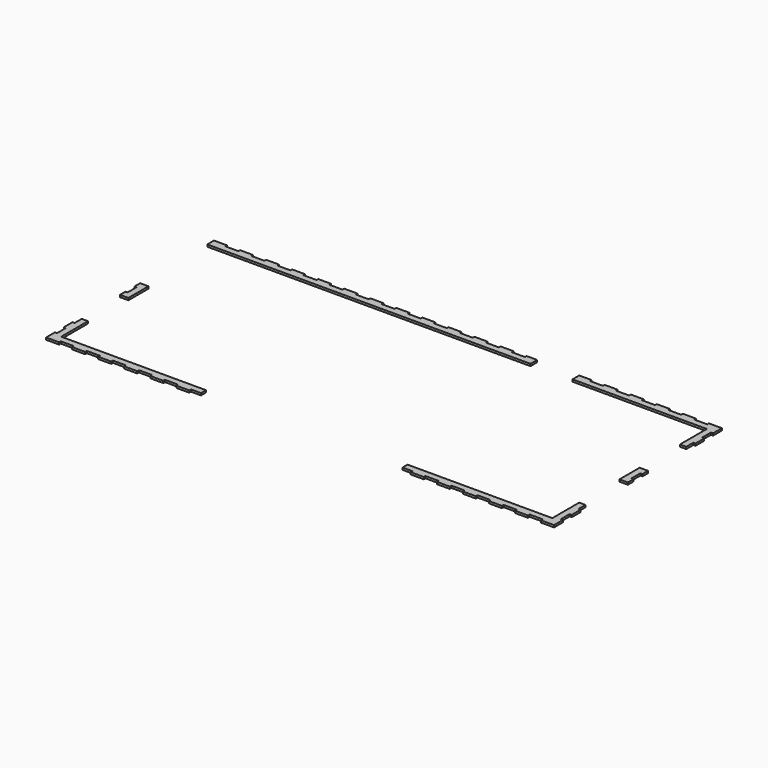
from build123d import *

# Parameters (mm, degrees)
F1_DEPTH = 3.175


# Not quite as in the source:
# - ends of sketch curves that miss each other by under 0.0002 mm in the source are joined


with BuildPart() as f1:
    # F0 (on Top) → F1 (new body)
    with BuildSketch(Plane.XY):
        Polygon((168.275, 158.75), (168.275, 146.05), (371.475, 146.05), (371.475, 95.25), (381, 95.25), (381, 108.618420812), (384.175, 108.618420812), (384.175, 125.328947208), (381, 125.328947208), (381, 142.039473604), (384.175, 142.039473604), (384.175, 155.575), (384.175004318, 158.75), (364.473722156, 158.75), (364.473722156, 155.575), (344.772439994, 155.575), (344.772439994, 158.75), (325.071157832, 158.75), (325.071157832, 155.575), (305.36987567, 155.575), (305.36987567, 158.75), (285.668593508, 158.75), (285.668593508, 155.575), (268.605, 155.575), (265.967311346, 155.575), (265.967311346, 158.75), (246.266029184, 158.75), (246.266029184, 155.575), (226.564747022, 155.575), (226.564747022, 158.75), (206.86346486, 158.75), (206.86346486, 155.575), (187.162182698, 155.575), (187.162182698, 158.75), align=None)
    extrude(amount=F1_DEPTH)


with BuildPart() as f1b:
    # F0 (on Top) → F1, piece 2 (new body)
    with BuildSketch(Plane.XY):
        Polygon((-364.473717838, 158.75), (-384.175, 158.75), (-384.175, 146.05), (-371.475, 146.05), (-317.7820146084, 146.05), (104.775, 146.05), (104.775, 158.75), (88.655771888, 158.75), (88.655771888, 155.575), (68.954489726, 155.575), (68.954489726, 158.75), (49.253207564, 158.75), (49.253207564, 155.575), (29.551925402, 155.575), (29.551925402, 158.75), (9.85064324, 158.75), (9.85064324, 155.575), (-9.850638922, 155.575), (-9.850638922, 158.75), (-29.551921084, 158.75), (-29.551921084, 155.575), (-49.253203246, 155.575), (-49.253203246, 158.75), (-68.954485408, 158.75), (-68.954485408, 155.575), (-88.65576757, 155.575), (-88.65576757, 158.75), (-108.357049732, 158.75), (-108.357049732, 155.575), (-128.058331894, 155.575), (-128.058331894, 158.75), (-147.759614056, 158.75), (-147.759614056, 155.575), (-167.460896218, 155.575), (-167.460896218, 158.75), (-187.16217838, 158.75), (-187.16217838, 155.575), (-206.863460542, 155.575), (-206.863460542, 158.75), (-226.564742704, 158.75), (-226.564742704, 155.575), (-246.266024866, 155.575), (-246.266024866, 158.75), (-265.967307028, 158.75), (-265.967307028, 155.575), (-285.66858919, 155.575), (-285.66858919, 158.75), (-305.369871352, 158.75), (-305.369871352, 155.575), (-325.071153514, 155.575), (-325.071153514, 158.75), (-344.772435676, 158.75), (-344.772435676, 155.575), (-364.473717838, 155.575), align=None)
    extrude(amount=F1_DEPTH)


with BuildPart() as f1c:
    # F0 (on Top) → F1, piece 3 (new body)
    with BuildSketch(Plane.XY):
        Polygon((-371.475, -19.05), (-371.475, 19.05), (-384.175, 19.05), (-384.175, 8.355262436), (-381, 8.355262436), (-381, -8.35526396), (-384.175, -8.35526396), (-384.175, -19.05), align=None)
    extrude(amount=F1_DEPTH)


with BuildPart() as f1d:
    # F0 (on Top) → F1, piece 4 (new body)
    with BuildSketch(Plane.XY):
        Polygon((-371.475, -146.05), (-371.475, -95.25), (-381, -95.25), (-381, -108.618422336), (-384.175, -108.618422336), (-384.175, -125.328948732), (-381, -125.328948732), (-381, -142.039475128), (-384.175, -142.039475128), (-384.175, -158.750001524), (-381, -158.750001524), (-364.473717838, -158.75), (-364.473717838, -155.575), (-344.772435676, -155.575), (-344.772435676, -158.75), (-325.071153514, -158.75), (-325.071153514, -155.575), (-305.369871352, -155.575), (-305.369871352, -158.75), (-285.66858919, -158.75), (-285.66858919, -155.575), (-265.967307028, -155.575), (-265.967307028, -158.75), (-246.266024866, -158.75), (-246.266024866, -155.575), (-226.564742704, -155.575), (-226.564742704, -158.75), (-206.863460542, -158.75), (-206.863460542, -155.575), (-187.16217838, -155.575), (-187.16217838, -158.75), (-167.460896218, -158.75), (-167.460896218, -155.575), (-152.4, -155.575), (-152.4, -146.05), align=None)
    extrude(amount=F1_DEPTH)


with BuildPart() as f1e:
    # F0 (on Top) → F1, piece 5 (new body)
    with BuildSketch(Plane.XY):
        Polygon((384.175, 19.05), (371.475, 19.05), (371.475, -19.05), (384.175, -19.05), (384.175, -8.35526396), (381, -8.35526396), (381, 8.355262436), (384.175, 8.355262436), align=None)
    extrude(amount=F1_DEPTH)


with BuildPart() as f1f:
    # F0 (on Top) → F1, piece 6 (new body)
    with BuildSketch(Plane.XY):
        Polygon((371.475, -146.05), (152.4, -146.05), (152.4, -155.575), (167.460900536, -155.575), (167.460900536, -158.75), (187.162182698, -158.75), (187.162182698, -155.575), (206.86346486, -155.575), (206.86346486, -158.75), (226.564747022, -158.75), (226.564747022, -155.575), (246.266029184, -155.575), (246.266029184, -158.75), (265.967311346, -158.75), (265.967311346, -155.575), (285.668593508, -155.575), (285.668593508, -158.75), (305.36987567, -158.75), (305.36987567, -155.575), (325.071157832, -155.575), (325.071157832, -158.75), (344.772439994, -158.75), (344.772439994, -155.575), (364.473722156, -155.575), (364.473722156, -158.75), (381, -158.75), (384.175004318, -158.75), (384.175004318, -155.575), (384.175, -142.039475128), (381, -142.039475128), (381, -125.328948732), (384.175, -125.328948732), (384.175, -108.618422336), (381, -108.618422336), (381, -95.25), (371.475, -95.25), align=None)
    extrude(amount=F1_DEPTH)


solid = Compound([f1.part, f1b.part, f1c.part, f1d.part, f1e.part, f1f.part])
